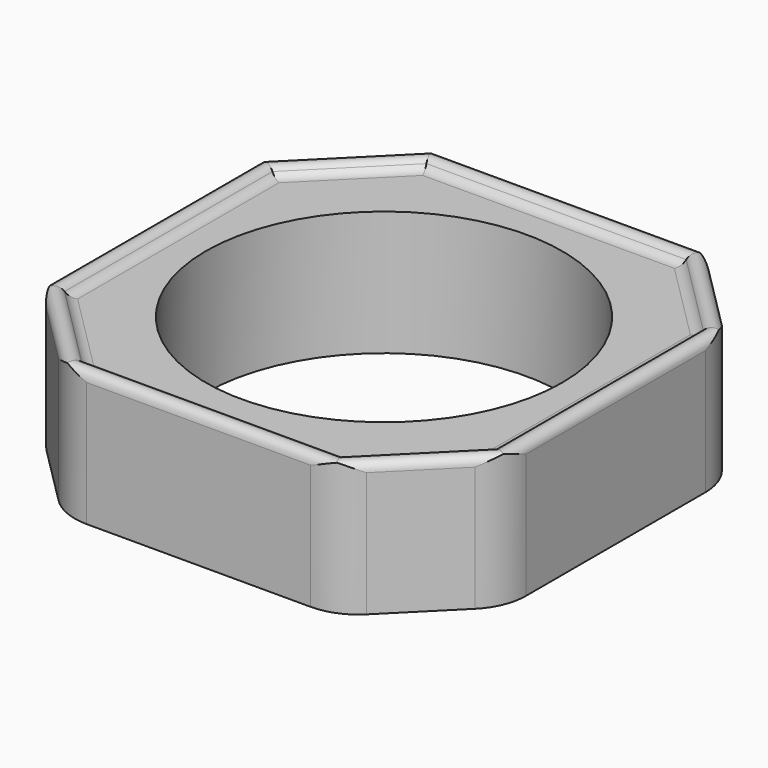
from build123d import *

# Parameters (mm, degrees)
F0_R        = 15
F1_DEPTH    = 10.5
F3_R        = 0.75
F5_R        = 1
F6_T1_DEPTH = 20.8553390593


# Not quite as in the source:
# - a fillet or chamfer that OpenCascade refuses, or shapes differently, is made with other operations: its cross-section is extruded or revolved along the edge and cut away or added


with BuildPart() as f1:
    # F0 (on Top) → F1 (new body)
    with BuildSketch(Plane.XY):
        Polygon((-11.5, -19.5), (11.5, -19.5), (19.5, -11.5), (19.5, 11.5), (11.5, 19.5), (-11.5, 19.5), (-19.5, 11.5), (-19.5, -11.5), align=None)
        Circle(F0_R, mode=Mode.SUBTRACT)
    extrude(amount=F1_DEPTH)

    # F4: sweep along a path in F2
    with BuildLine(Plane.XY.offset(10.5)) as f4_path:
        Line((18.75, 11.1893398282), (18.75, -11.1893398282))
        Line((18.75, -11.1893398282), (11.1893398282, -18.75))
        Line((11.1893398282, -18.75), (-11.1893398282, -18.75))
        Line((-11.1893398282, -18.75), (-18.75, -11.1893398282))
        Line((-18.75, -11.1893398282), (-18.75, 11.1893398282))
        Line((-18.75, 11.1893398282), (-11.1893398282, 18.75))
        Line((-11.1893398282, 18.75), (11.1893398282, 18.75))
        Line((11.1893398282, 18.75), (18.75, 11.1893398282))
    # F3 (on Front) → F4 (sweep)
    with BuildSketch(Plane.XZ):
        with Locations((18.75, 10.5)):
            Circle(F3_R)
    sweep(path=f4_path.line, transition=Transition.RIGHT)

    # F5
    f5_edges = [f1.edges().sort_by_distance(p)[0] for p in [
        (18, 0, 10.5),
        (14.43934, -14.43934, 10.5),
        (0, -18, 10.5),
        (-14.43934, -14.43934, 10.5),
        (-18, 0, 10.5),
        (-14.43934, 14.43934, 10.5),
        (0, 18, 10.5),
        (14.43934, 14.43934, 10.5),
    ]]
    fillet(f5_edges, radius=F5_R)

    # F6: fillet of radius 5 on 8 edges, made by hand

    # F6_s2 → F6_t1 (cut)
    with BuildSketch(Plane.XY.offset(-5.1776695297)):
        with BuildLine():
            ThreePointArc((-18.0355339059, -12.9644660941), (-19.1193976626, -11.34234935), (-19.5, -9.4289321881))
            Line((-19.5, -9.4289321881), (-19.5, -11.5))
            Line((-19.5, -11.5), (-18.0355339059, -12.9644660941))
        make_face()
        with BuildLine():
            ThreePointArc((-9.4289321881, -19.5), (-11.34234935, -19.1193976626), (-12.9644660941, -18.0355339059))
            Line((-12.9644660941, -18.0355339059), (-11.5, -19.5))
            Line((-11.5, -19.5), (-9.4289321881, -19.5))
        make_face()
        with BuildLine():
            ThreePointArc((9.4289321881, -19.5), (11.34234935, -19.1193976626), (12.9644660941, -18.0355339059))
            Line((12.9644660941, -18.0355339059), (11.5, -19.5))
            Line((11.5, -19.5), (9.4289321881, -19.5))
        make_face()
        with BuildLine():
            ThreePointArc((18.0355339059, -12.9644660941), (19.1193976626, -11.34234935), (19.5, -9.4289321881))
            Line((19.5, -9.4289321881), (19.5, -11.5))
            Line((19.5, -11.5), (18.0355339059, -12.9644660941))
        make_face()
        with BuildLine():
            ThreePointArc((-9.4289321881, 19.5), (-11.34234935, 19.1193976626), (-12.9644660941, 18.0355339059))
            Line((-12.9644660941, 18.0355339059), (-11.5, 19.5))
            Line((-11.5, 19.5), (-9.4289321881, 19.5))
        make_face()
        with BuildLine():
            ThreePointArc((-19.5, 9.4289321881), (-19.1193976626, 11.34234935), (-18.0355339059, 12.9644660941))
            Line((-18.0355339059, 12.9644660941), (-19.5, 11.5))
            Line((-19.5, 11.5), (-19.5, 9.4289321881))
        make_face()
        with BuildLine():
            ThreePointArc((12.9644660941, 18.0355339059), (11.34234935, 19.1193976626), (9.4289321881, 19.5))
            Line((9.4289321881, 19.5), (11.5, 19.5))
            Line((11.5, 19.5), (12.9644660941, 18.0355339059))
        make_face()
        with BuildLine():
            ThreePointArc((19.5, 9.4289321881), (19.1193976626, 11.34234935), (18.0355339059, 12.9644660941))
            Line((18.0355339059, 12.9644660941), (19.5, 11.5))
            Line((19.5, 11.5), (19.5, 9.4289321881))
        make_face()
    extrude(amount=F6_T1_DEPTH, mode=Mode.SUBTRACT)


solid = f1.part
